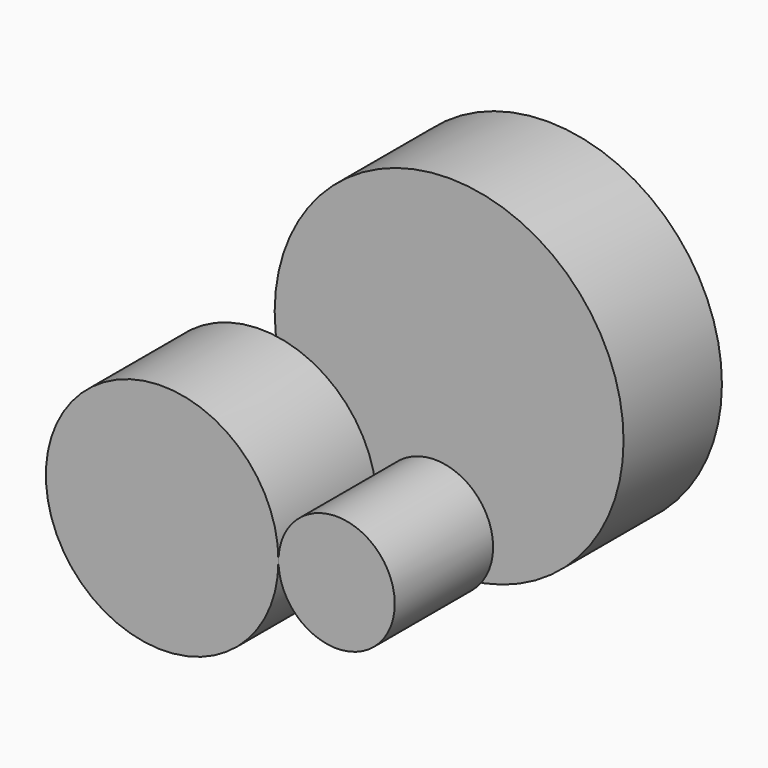
from build123d import *

# Parameters (mm, degrees)
F0_R     = 70
F1_DEPTH = 148
F2_R     = 140
F3_DEPTH = 148
F5_DEPTH = 148


# Not quite as in the source:
# - a feature of the source that left no trace in its solid (it failed there, or was rolled back) is left out


with BuildPart() as f1:
    # F0 (on Front) → F1 (new body)
    with BuildSketch(Plane.XZ):
        Circle(F0_R)
    extrude(amount=F1_DEPTH)


with BuildPart() as f3:
    # F2 (on Front) → F3 (new body)
    with BuildSketch(Plane.XZ):
        with Locations((-210, 0)):
            Circle(F2_R)
    extrude(amount=F3_DEPTH)


with BuildPart() as f5:
    # F4 (on Front) → F5 (new body)
    with BuildSketch(Plane.XZ):
        with BuildLine():
            ThreePointArc((-153.2385760506, 40.9651162727), (-276.6081814662, -21.5255699523), (-140, 0))
            ThreePointArc((-140, 0), (-143.3918185338, 21.5255699523), (-153.2385760506, 40.9651162727))
        make_face()
    extrude(amount=-F5_DEPTH)


with BuildPart() as f5b:
    # F4 (on Front) → F5, piece 2 (new body)
    with BuildSketch(Plane.XZ):
        with BuildLine():
            ThreePointArc((227.0456952089, 163.8604659066), (-47.5310151267, 363.6850101504), (-153.2385760506, 40.9651162727))
            ThreePointArc((-153.2385760506, 40.9651162727), (81.6224055444, -35.9640783372), (227.0456952089, 163.8604659066))
        make_face()
    extrude(amount=-F5_DEPTH)


solid = Compound([f1.part, f3.part, f5.part, f5b.part])
